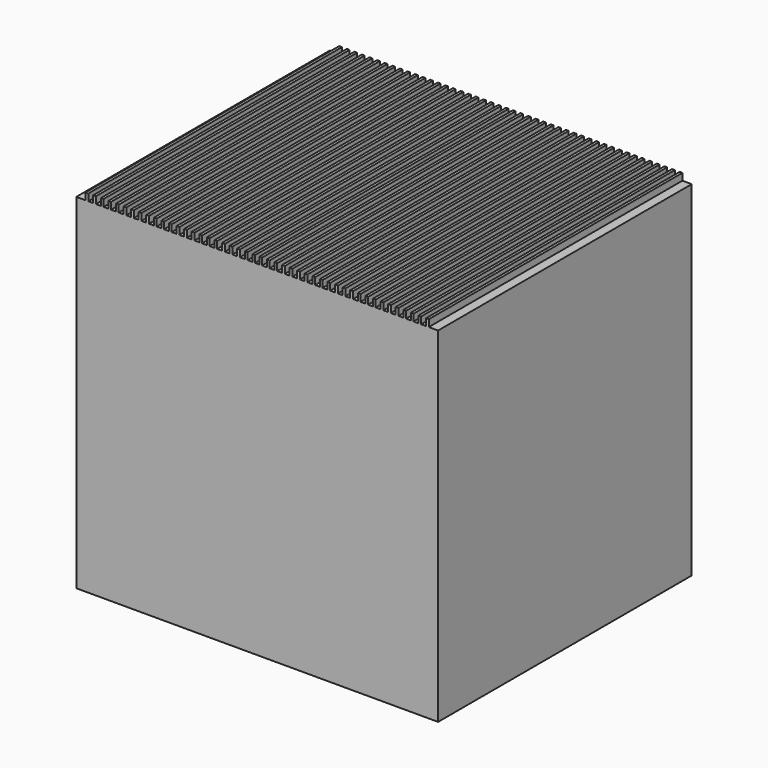
from build123d import *

# Parameters (mm, degrees)
F2_W         = 10.5
F2_H         = 9.2
F3_DEPTH     = 10
F4_W         = 0.08
F4_H         = 9.2
F5_DEPTH     = 0.2
F6_TEXT_SIZE = 10.3442195622
F7_DEPTH     = 2


# Not quite as in the source:
# - Text() gives the source's letters only with a copy of the font that has no kerning and outlines rounded to 1/6400 em; it was checked with that copy


with BuildPart() as f3:
    # F2 (on Top) → F3 (new body)
    with BuildSketch(Plane.XY):
        Rectangle(F2_W, F2_H)
    extrude(amount=F3_DEPTH)

    # F4 (on face) → F5 (join)
    with BuildSketch(Plane.XY.offset(10)):
        with Locations((0.1, 0)):
            Rectangle(F4_W, F4_H)
        with Locations((0.32, 0)):
            Rectangle(F4_W, F4_H)
        with Locations((0.54, 0)):
            Rectangle(F4_W, F4_H)
        with Locations((0.76, 0)):
            Rectangle(F4_W, F4_H)
        with Locations((0.98, 0)):
            Rectangle(F4_W, F4_H)
        with Locations((1.2, 0)):
            Rectangle(F4_W, F4_H)
        with Locations((1.42, 0)):
            Rectangle(F4_W, F4_H)
        with Locations((1.64, 0)):
            Rectangle(F4_W, F4_H)
        with Locations((1.86, 0)):
            Rectangle(F4_W, F4_H)
        with Locations((2.08, 0)):
            Rectangle(F4_W, F4_H)
        with Locations((2.3, 0)):
            Rectangle(F4_W, F4_H)
        with Locations((2.52, 0)):
            Rectangle(F4_W, F4_H)
        with Locations((2.74, 0)):
            Rectangle(F4_W, F4_H)
        with Locations((2.96, 0)):
            Rectangle(F4_W, F4_H)
        with Locations((3.18, 0)):
            Rectangle(F4_W, F4_H)
        with Locations((3.4, 0)):
            Rectangle(F4_W, F4_H)
        with Locations((3.62, 0)):
            Rectangle(F4_W, F4_H)
        with Locations((3.84, 0)):
            Rectangle(F4_W, F4_H)
        with Locations((4.06, 0)):
            Rectangle(F4_W, F4_H)
        with Locations((4.28, 0)):
            Rectangle(F4_W, F4_H)
        with Locations((4.5, 0)):
            Rectangle(F4_W, F4_H)
        with Locations((4.72, 0)):
            Rectangle(F4_W, F4_H)
        with Locations((4.94, 0)):
            Rectangle(F4_W, F4_H)
        with Locations((-0.32, 0)):
            Rectangle(F4_W, F4_H)
        with Locations((-0.1, 0)):
            Rectangle(F4_W, F4_H)
        with Locations((-3.84, 0)):
            Rectangle(F4_W, F4_H)
        with Locations((-2.08, 0)):
            Rectangle(F4_W, F4_H)
        with Locations((-2.96, 0)):
            Rectangle(F4_W, F4_H)
        with Locations((-1.42, 0)):
            Rectangle(F4_W, F4_H)
        with Locations((-1.64, 0)):
            Rectangle(F4_W, F4_H)
        with Locations((-1.2, 0)):
            Rectangle(F4_W, F4_H)
        with Locations((-4.06, 0)):
            Rectangle(F4_W, F4_H)
        with Locations((-4.94, 0)):
            Rectangle(F4_W, F4_H)
        with Locations((-2.74, 0)):
            Rectangle(F4_W, F4_H)
        with Locations((-0.76, 0)):
            Rectangle(F4_W, F4_H)
        with Locations((-4.72, 0)):
            Rectangle(F4_W, F4_H)
        with Locations((-3.62, 0)):
            Rectangle(F4_W, F4_H)
        with Locations((-2.3, 0)):
            Rectangle(F4_W, F4_H)
        with Locations((-3.18, 0)):
            Rectangle(F4_W, F4_H)
        with Locations((-2.52, 0)):
            Rectangle(F4_W, F4_H)
        with Locations((-4.28, 0)):
            Rectangle(F4_W, F4_H)
        with Locations((-3.4, 0)):
            Rectangle(F4_W, F4_H)
        with Locations((-0.98, 0)):
            Rectangle(F4_W, F4_H)
        with Locations((-4.5, 0)):
            Rectangle(F4_W, F4_H)
        with Locations((-1.86, 0)):
            Rectangle(F4_W, F4_H)
        with Locations((-0.54, 0)):
            Rectangle(F4_W, F4_H)
    extrude(amount=F5_DEPTH)

    # F6 (on face) → F7 (cut)
    with BuildSketch(Plane(origin=(0, 0, 0), x_dir=(1, 0, 0), z_dir=(0, 0, -1))):
        with Locations((-2.895952377, -3.7031605607)):
            Text('1', F6_TEXT_SIZE, font='Open Sans', font_style=FontStyle.BOLD, text_align=(TextAlign.LEFT, TextAlign.BOTTOM))
    extrude(amount=-F7_DEPTH, mode=Mode.SUBTRACT)


solid = f3.part
